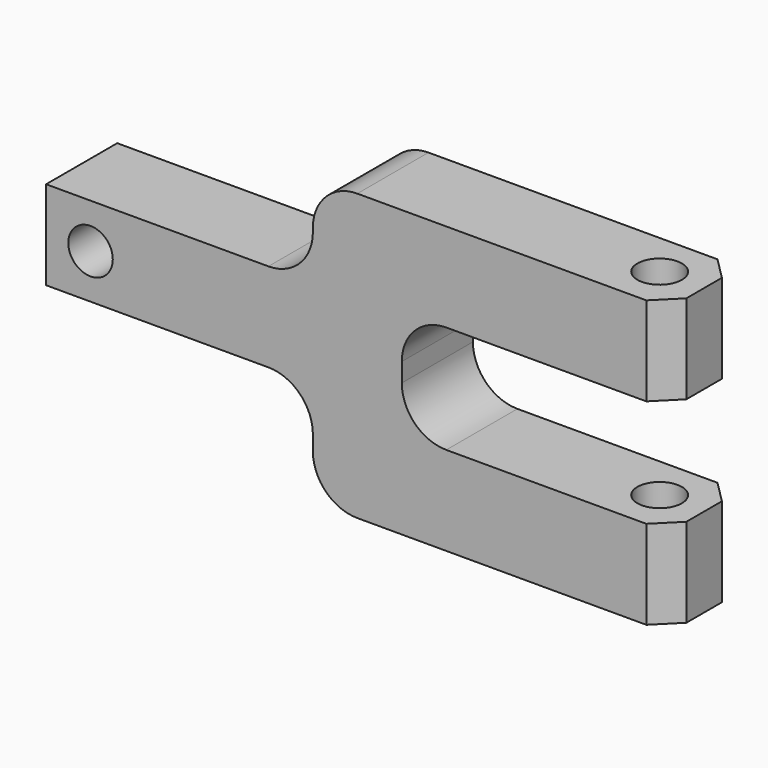
from build123d import *

# Parameters (mm, degrees)
F0_R     = 6.35
F1_DEPTH = 12.7
F2_R     = 6.35
F3_DEPTH = 25.4
F4_R     = 6.35
F5_DEPTH = 25.4
F6_SIZE  = 6.35


# Not quite as in the source:
# - a feature names something its author has since deleted; it is built from what else it names


with BuildPart() as f1:
    # F0 (on Front) → F1 (new body, symmetric)
    with BuildSketch(Plane.XZ):
        with BuildLine():
            Line((-127, -12.7), (-63.5, -12.7))
            ThreePointArc((-63.5, -12.7), (-54.5197438789, -16.4197438789), (-50.8, -25.4))
            Line((-50.8, -25.4), (-50.8, -29.6333387181))
            ThreePointArc((-50.8, -29.6333387181), (-47.0802561211, -38.6135948391), (-38.1, -42.3333387181))
            Line((-38.1, -42.3333387181), (50.8, -42.3333387181))
            Line((50.8, -42.3333387181), (50.8, -16.9333387181))
            Line((50.8, -16.9333387181), (-12.7, -16.9333387181))
            ThreePointArc((-12.7, -16.9333387181), (-21.6802561211, -13.2135948391), (-25.4, -4.2333387181))
            Line((-25.4, -4.2333387181), (-25.4, 1.1545434965))
            ThreePointArc((-25.4, 1.1545434965), (-21.6802561211, 10.1347996175), (-12.7, 13.8545434965))
            Line((-12.7, 13.8545434965), (50.8, 13.8545434965))
            Line((50.8, 13.8545434965), (50.8, 39.2545434965))
            Line((50.8, 39.2545434965), (-38.1, 39.2545434965))
            ThreePointArc((-38.1, 39.2545434965), (-47.0802561211, 35.5347996175), (-50.8, 26.5545434965))
            Line((-50.8, 26.5545434965), (-50.8, 25.4))
            ThreePointArc((-50.8, 25.4), (-54.5197438789, 16.4197438789), (-63.5, 12.7))
            Line((-63.5, 12.7), (-127, 12.7))
            Line((-127, 12.7), (-127, -12.7))
        make_face()
        with Locations((-114.3, 0)):
            Circle(F0_R, mode=Mode.SUBTRACT)
    extrude(amount=F1_DEPTH, both=True)

    # F2 (on face) → F3 (cut)
    with BuildSketch(Plane(origin=(0, 0, 13.8545434965), x_dir=(1, 0, 0), z_dir=(0, 0, -1))):
        with Locations((38.1, 0)):
            Circle(F2_R)
    extrude(amount=-F3_DEPTH, mode=Mode.SUBTRACT)

    # F4 (on face) → F5 (cut)
    with BuildSketch(Plane(origin=(0, 0, -42.3333387181), x_dir=(1, 0, 0), z_dir=(0, 0, -1))):
        with Locations((38.1, 0)):
            Circle(F4_R)
    extrude(amount=-F5_DEPTH, mode=Mode.SUBTRACT)

    # F6
    f6_edges = [f1.edges().sort_by_distance(p)[0] for p in [
        (50.8, -12.7, -29.633339),
        (50.8, 12.7, -29.633339),
        (50.8, -12.7, 26.554543),
        (50.8, 12.7, 26.554543),
    ]]
    chamfer(f6_edges, length=F6_SIZE)


solid = f1.part
